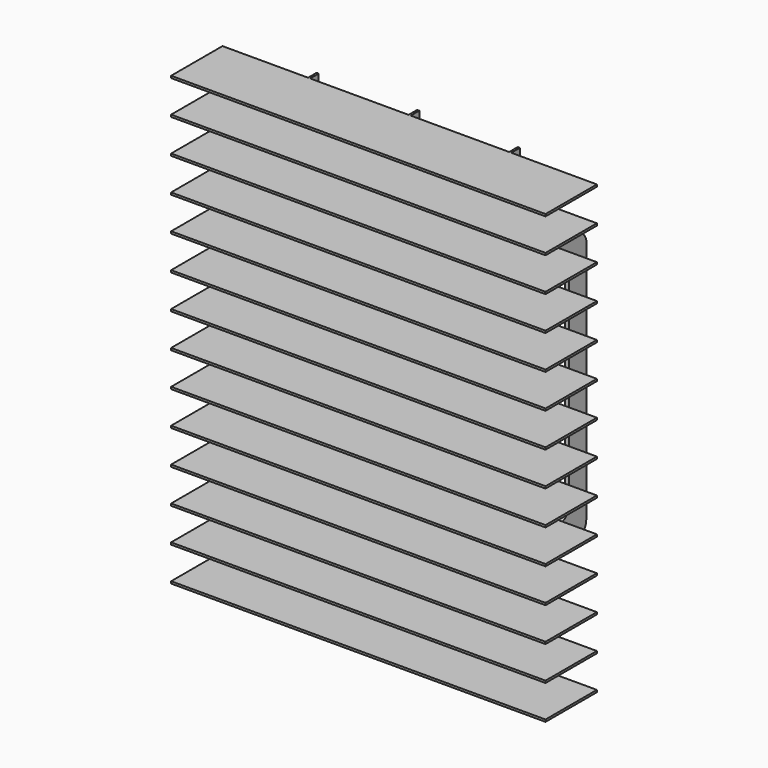
from build123d import *

# Parameters (mm, degrees)
F0_W     = 350
F0_H     = 2
F1_DEPTH = 60
F2_W     = 2
F2_H     = 20
F3_DEPTH = 450
F6_DEPTH = 2
F8_DEPTH = 4


with BuildPart() as f1:
    # F0 (on Front) → F1 (new body)
    with BuildSketch(Plane.XZ):
        with Locations((-175, 417)):
            Rectangle(F0_W, F0_H)
    extrude(amount=F1_DEPTH)

    # F2 (on face) → F3 (join)
    with BuildSketch(Plane.XY.offset(418)):
        with Locations((-269, 0)):
            Rectangle(F2_W, F2_H)
        with Locations((-81, 0)):
            Rectangle(F2_W, F2_H)
        with Locations((-175, 0)):
            Rectangle(F2_W, F2_H)
    extrude(amount=-F3_DEPTH)

    # F5 (on face) → F6 (join, symmetric)
    with BuildSketch(Plane(origin=(-270, 0, 0), x_dir=(0, -1, 0), z_dir=(-1, 0, 0))):
        with BuildLine():
            Line((-10, 318), (-70, 318))
            Line((-70, 318), (-80, 318))
            ThreePointArc((-80, 318), (-87.0710678119, 315.0710678119), (-90, 308))
            Line((-90, 308), (-90, 78))
            ThreePointArc((-90, 78), (-87.0710678119, 70.9289321881), (-80, 68))
            Line((-80, 68), (-70, 68))
            Line((-70, 68), (-10, 68))
            Line((-10, 68), (-10, 88))
            Line((-10, 88), (-60, 88))
            ThreePointArc((-60, 88), (-67.0710678119, 90.9289321881), (-70, 98))
            Line((-70, 98), (-70, 288))
            ThreePointArc((-70, 288), (-67.0710678119, 295.0710678119), (-60, 298))
            Line((-60, 298), (-10, 298))
            Line((-10, 298), (-10, 318))
        make_face()
    extrude(amount=F6_DEPTH, both=True)


with BuildPart() as f1b:
    # F0 (on Front) → F1, piece 2 (new body)
    with BuildSketch(Plane.XZ):
        with Locations((-175, 385)):
            Rectangle(F0_W, F0_H)
    extrude(amount=F1_DEPTH)


with BuildPart() as f1c:
    # F0 (on Front) → F1, piece 3 (new body)
    with BuildSketch(Plane.XZ):
        with Locations((-175, 353)):
            Rectangle(F0_W, F0_H)
    extrude(amount=F1_DEPTH)


with BuildPart() as f1d:
    # F0 (on Front) → F1, piece 4 (new body)
    with BuildSketch(Plane.XZ):
        with Locations((-175, 321)):
            Rectangle(F0_W, F0_H)
    extrude(amount=F1_DEPTH)


with BuildPart() as f1e:
    # F0 (on Front) → F1, piece 5 (new body)
    with BuildSketch(Plane.XZ):
        with Locations((-175, 289)):
            Rectangle(F0_W, F0_H)
    extrude(amount=F1_DEPTH)


with BuildPart() as f1f:
    # F0 (on Front) → F1, piece 6 (new body)
    with BuildSketch(Plane.XZ):
        with Locations((-175, 257)):
            Rectangle(F0_W, F0_H)
    extrude(amount=F1_DEPTH)


with BuildPart() as f1g:
    # F0 (on Front) → F1, piece 7 (new body)
    with BuildSketch(Plane.XZ):
        with Locations((-175, 225)):
            Rectangle(F0_W, F0_H)
    extrude(amount=F1_DEPTH)


with BuildPart() as f1h:
    # F0 (on Front) → F1, piece 8 (new body)
    with BuildSketch(Plane.XZ):
        with Locations((-175, 193)):
            Rectangle(F0_W, F0_H)
    extrude(amount=F1_DEPTH)


with BuildPart() as f1i:
    # F0 (on Front) → F1, piece 9 (new body)
    with BuildSketch(Plane.XZ):
        with Locations((-175, 161)):
            Rectangle(F0_W, F0_H)
    extrude(amount=F1_DEPTH)


with BuildPart() as f1j:
    # F0 (on Front) → F1, piece 10 (new body)
    with BuildSketch(Plane.XZ):
        with Locations((-175, 129)):
            Rectangle(F0_W, F0_H)
    extrude(amount=F1_DEPTH)


with BuildPart() as f1k:
    # F0 (on Front) → F1, piece 11 (new body)
    with BuildSketch(Plane.XZ):
        with Locations((-175, 97)):
            Rectangle(F0_W, F0_H)
    extrude(amount=F1_DEPTH)


with BuildPart() as f1l:
    # F0 (on Front) → F1, piece 12 (new body)
    with BuildSketch(Plane.XZ):
        with Locations((-175, 65)):
            Rectangle(F0_W, F0_H)
    extrude(amount=F1_DEPTH)


with BuildPart() as f1m:
    # F0 (on Front) → F1, piece 13 (new body)
    with BuildSketch(Plane.XZ):
        with Locations((-175, 33)):
            Rectangle(F0_W, F0_H)
    extrude(amount=F1_DEPTH)


with BuildPart() as f1n:
    # F0 (on Front) → F1, piece 14 (new body)
    with BuildSketch(Plane.XZ):
        with Locations((-175, 1)):
            Rectangle(F0_W, F0_H)
    extrude(amount=F1_DEPTH)


with BuildPart() as f8:
    # F7 (on face) → F8 (new body)
    with BuildSketch(Plane(origin=(-82, 0, 0), x_dir=(0, -1, 0), z_dir=(-1, 0, 0))):
        with BuildLine():
            Line((-10, 298.2498407364), (-10, 318.1632757187))
            Line((-10, 318.1632757187), (-78.7753984332, 318.1632757187))
            ThreePointArc((-78.7753984332, 318.1632757187), (-86.1493487568, 315.4987990699), (-90.1169553399, 308.736205101))
            Line((-90.1169553399, 308.736205101), (-90.1169553399, 78.6898061633))
            ThreePointArc((-90.1169553399, 78.6898061633), (-87.4254689451, 71.609182036), (-80.7102024555, 68.1042522192))
            Line((-80.7102024555, 68.1042522192), (-10, 68.1042522192))
            Line((-10, 68.1042522192), (-10, 88.0431681871))
            Line((-10, 88.0431681871), (-59.2116527259, 88.0431681871))
            ThreePointArc((-59.2116527259, 88.0431681871), (-66.5650380478, 90.9297800306), (-69.9910148978, 98.0478897691))
            Line((-69.9910148978, 98.0478897691), (-69.9910148978, 288.1482243538))
            ThreePointArc((-69.9910148978, 288.1482243538), (-67.5769986798, 294.8224551486), (-61.3620281219, 298.2498407364))
            Line((-61.3620281219, 298.2498407364), (-10, 298.2498407364))
        make_face()
    extrude(amount=F8_DEPTH)


solid = Compound([f1.part, f1b.part, f1c.part, f1d.part, f1e.part, f1f.part, f1g.part, f1h.part, f1i.part, f1j.part, f1k.part, f1l.part, f1m.part, f1n.part, f8.part])
